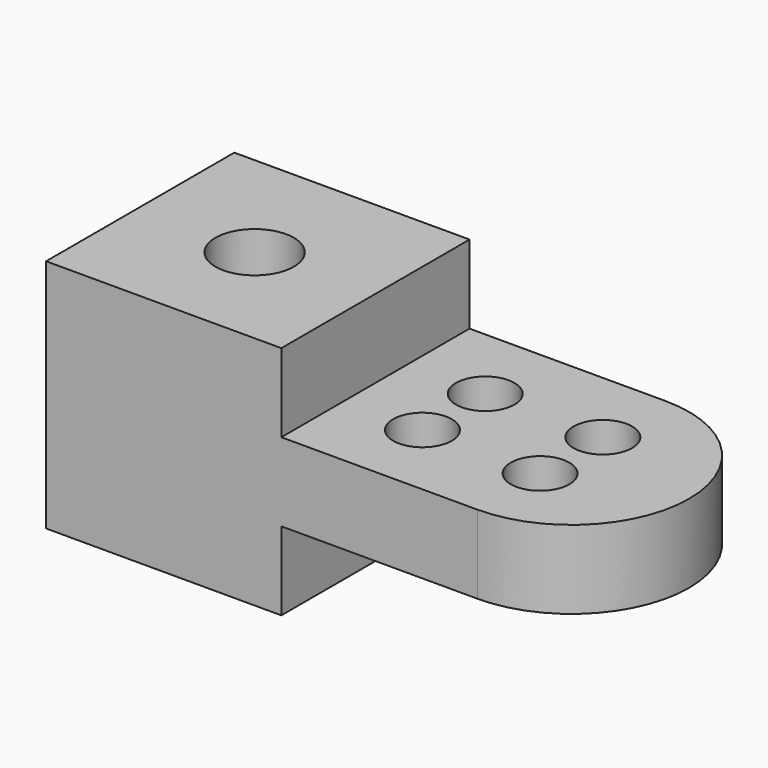
from build123d import *

# Parameters (mm, degrees)
F1_DEPTH = 38.1
F3_DEPTH = 12.7
F4_R     = 6.35
F4_R_2   = 4.745300615
F5_DEPTH = 38.101


# Not quite as in the source:
# - a feature names something its author has since deleted; it is built from what else it names


with BuildPart() as f1:
    # F0 (on Front) → F1 (new body)
    with BuildSketch(Plane.XZ):
        Polygon((0, 38.1), (0, 0), (38.1, 0), (38.1, 12.7), (69.85, 12.7), (69.85, 25.4), (38.1, 25.4), (38.1, 38.1), align=None)
    extrude(amount=F1_DEPTH)

    # F2 (on face) → F3 (join)
    with BuildSketch(Plane.XY.offset(25.4)):
        with BuildLine():
            Line((69.85, 0), (69.85, -38.1))
            ThreePointArc((69.85, -38.1), (88.9, -19.05), (69.85, 0))
        make_face()
    extrude(amount=-F3_DEPTH)

    # F4 (on face) → F5 (cut, through all)
    with BuildSketch(Plane.XY.offset(38.1)):
        with Locations((19.05, -19.6927841753)):
            Circle(F4_R)
        with Locations((50.8, -12.7)):
            Circle(F4_R_2)
        with Locations((50.8, -25.4)):
            Circle(F4_R_2)
        with Locations((69.85, -25.4)):
            Circle(F4_R_2)
        with Locations((69.85, -12.7)):
            Circle(F4_R_2)
    extrude(amount=-F5_DEPTH, mode=Mode.SUBTRACT)


solid = f1.part
